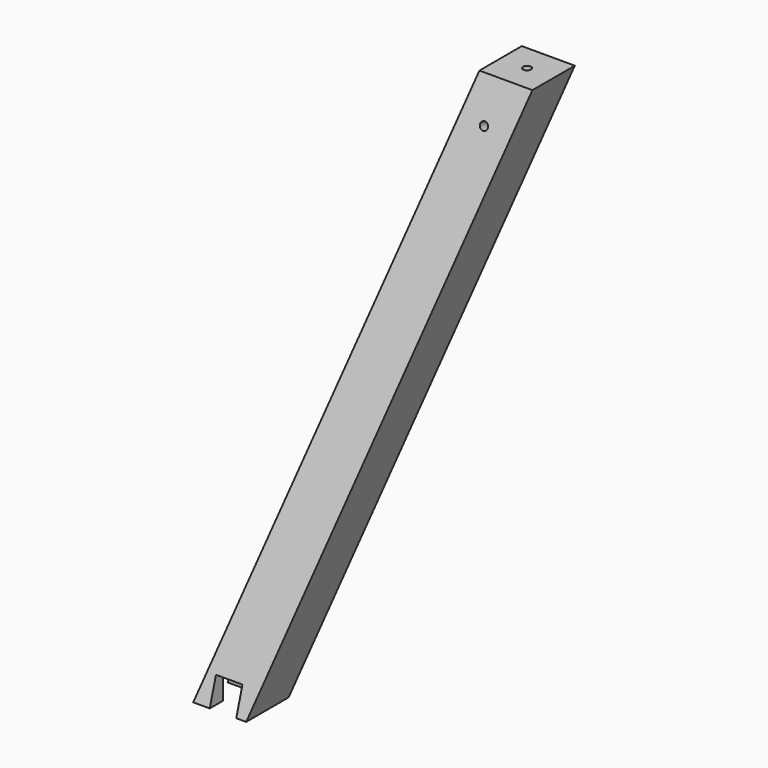
from build123d import *

# Parameters (mm, degrees)
F0_W      = 40
F0_H      = 40
F2_W      = 40
F2_H      = 40
F4_R      = 3
F5_DEPTH  = 12
F6_R      = 3
F7_DEPTH  = 12
F8_R      = 3
F9_DEPTH  = 12
F11_W     = 20
F11_H     = 20
F12_DEPTH = 32.5
F14_W     = 20
F14_H     = 20
F15_DEPTH = 32.5
F16_R     = 3
F17_DEPTH = 4
F18_R     = 3
F19_DEPTH = 4


with BuildPart() as f3:
    # F0 (on Top) → F3 section 0
    with BuildSketch(Plane.XY):
        Rectangle(F0_W, F0_H)
    # F2 (on offset) → F3 section 1
    with BuildSketch(Plane.XY.offset(410)):
        with Locations((120, 120)):
            Rectangle(F2_W, F2_H)
    loft()

    # F4 (on face) → F5 (cut)
    with BuildSketch(Plane(origin=(-18.4219178082, 0, 5.3917808219), x_dir=(0, -1, 0), z_dir=(-0.959737407, 0, 0.2808987533))):
        with Locations((-112.0100207019, 390.3822122005)):
            Circle(F4_R)
    extrude(amount=-F5_DEPTH, mode=Mode.SUBTRACT)

    # F6 (on face) → F7 (cut)
    with BuildSketch(Plane(origin=(0, -18.4219178082, 5.3917808219), x_dir=(1, 0, 0), z_dir=(0, -0.959737407, 0.2808987533))):
        with Locations((110.461897094, 390.3822122005)):
            Circle(F6_R)
    extrude(amount=-F7_DEPTH, mode=Mode.SUBTRACT)

    # F8 (on face) → F9 (cut)
    with BuildSketch(Plane.XY.offset(410)):
        with Locations((120, 120)):
            Circle(F8_R)
    extrude(amount=-F9_DEPTH, mode=Mode.SUBTRACT)

    # F11 (on offset) → F12 (cut)
    with BuildSketch(Plane.YZ.offset(-20)):
        with Locations((2.5, 10)):
            Rectangle(F11_W, F11_H)
    extrude(amount=F12_DEPTH, mode=Mode.SUBTRACT)

    # F14 (on offset) → F15 (cut)
    with BuildSketch(Plane.XZ.offset(20)):
        with Locations((2.5, 10)):
            Rectangle(F14_W, F14_H)
    extrude(amount=-F15_DEPTH, mode=Mode.SUBTRACT)

    # F16 (on face) → F17 (cut)
    with BuildSketch(Plane.XZ.offset(-12.5)):
        with Locations((2.5, 10)):
            Circle(F16_R)
    extrude(amount=-F17_DEPTH, mode=Mode.SUBTRACT)

    # F18 (on face) → F19 (cut)
    with BuildSketch(Plane(origin=(12.5, 0, 0), x_dir=(0, -1, 0), z_dir=(-1, 0, 0))):
        with Locations((-2.5, 10)):
            Circle(F18_R)
    extrude(amount=-F19_DEPTH, mode=Mode.SUBTRACT)


solid = f3.part
